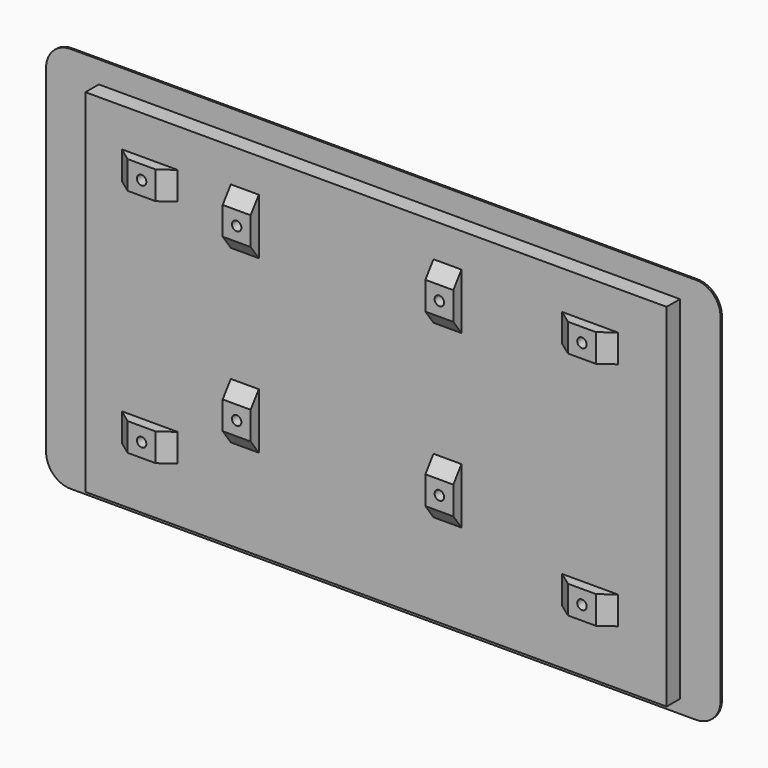
from build123d import *

# Parameters (mm, degrees)
F0_W     = 166.3
F0_H     = 100.7
F0_W_2   = 154.8
F0_H_2   = 87.4
F0_W_3   = 8
F0_H_3   = 8
F0_R     = 1.35
F1_DEPTH = 0.5
F2_DEPTH = 4.8
F3_DEPTH = 7.7
F4_SIZE2 = 2.89999
F4_SIZE  = 3.99999
F5_DEPTH = 0.51


# Not quite as in the source:
# - a fillet or chamfer is up to 0.001 mm smaller than in the source, because OpenCascade refuses the exact size


with BuildPart() as f1:
    # F0 (on Front) → F1 (new body)
    with BuildSketch(Plane.XZ):
        with BuildLine():
            Line((67.3, 73), (-111.7, 73))
            ThreePointArc((-111.7, 73), (-116.6497474683, 70.9497474683), (-118.7, 66))
            Line((-118.7, 66), (-118.7, -30.8))
            ThreePointArc((-118.7, -30.8), (-116.6497474683, -35.7497474683), (-111.7, -37.8))
            Line((-111.7, -37.8), (67.3, -37.8))
            ThreePointArc((67.3, -37.8), (72.2497474683, -35.7497474683), (74.3, -30.8))
            Line((74.3, -30.8), (74.3, 66))
            ThreePointArc((74.3, 66), (72.2497474683, 70.9497474683), (67.3, 73))
        make_face()
        with Locations((-20.45, 16.35)):
            Rectangle(F0_W, F0_H, mode=Mode.SUBTRACT)
        with Locations((-20.45, 16.35)):
            Rectangle(F0_W, F0_H)
        with Locations((-22.2, 18.6)):
            Rectangle(F0_W_2, F0_H_2, mode=Mode.SUBTRACT)
        with Locations((-22.2, 18.6)):
            Rectangle(F0_W_2, F0_H_2)
        with Locations((-85.2, -14.3)):
            Rectangle(F0_W_3, F0_H_3, mode=Mode.SUBTRACT)
        with Locations((-58, 0)):
            Rectangle(F0_W_3, F0_H_3, mode=Mode.SUBTRACT)
        with Locations((40.8, -14.3)):
            Rectangle(F0_W_3, F0_H_3, mode=Mode.SUBTRACT)
        Rectangle(F0_W_3, F0_H_3, mode=Mode.SUBTRACT)
        with Locations((-85.2, 51.7)):
            Rectangle(F0_W_3, F0_H_3, mode=Mode.SUBTRACT)
        with Locations((-58, 49)):
            Rectangle(F0_W_3, F0_H_3, mode=Mode.SUBTRACT)
        with Locations((0, 49)):
            Rectangle(F0_W_3, F0_H_3, mode=Mode.SUBTRACT)
        with Locations((40.8, 51.7)):
            Rectangle(F0_W_3, F0_H_3, mode=Mode.SUBTRACT)
        with Locations((-58, 49)):
            Rectangle(F0_W_3, F0_H_3)
        with Locations((-58, 49)):
            Circle(F0_R, mode=Mode.SUBTRACT)
        with Locations((-85.2, 51.7)):
            Rectangle(F0_W_3, F0_H_3)
        with Locations((-85.2, 51.7)):
            Circle(F0_R, mode=Mode.SUBTRACT)
        with Locations((40.8, 51.7)):
            Rectangle(F0_W_3, F0_H_3)
        with Locations((40.8, 51.7)):
            Circle(F0_R, mode=Mode.SUBTRACT)
        Rectangle(F0_W_3, F0_H_3)
        Circle(F0_R, mode=Mode.SUBTRACT)
        with Locations((40.8, -14.3)):
            Rectangle(F0_W_3, F0_H_3)
        with Locations((40.8, -14.3)):
            Circle(F0_R, mode=Mode.SUBTRACT)
        with Locations((0, 49)):
            Rectangle(F0_W_3, F0_H_3)
        with Locations((0, 49)):
            Circle(F0_R, mode=Mode.SUBTRACT)
        with Locations((-58, 0)):
            Rectangle(F0_W_3, F0_H_3)
        with Locations((-58, 0)):
            Circle(F0_R, mode=Mode.SUBTRACT)
        with Locations((-85.2, -14.3)):
            Rectangle(F0_W_3, F0_H_3)
        with Locations((-85.2, -14.3)):
            Circle(F0_R, mode=Mode.SUBTRACT)
        with Locations((0, 49)):
            Circle(F0_R)
        with Locations((40.8, 51.7)):
            Circle(F0_R)
        with Locations((40.8, -14.3)):
            Circle(F0_R)
        Circle(F0_R)
        with Locations((-58, 49)):
            Circle(F0_R)
        with Locations((-58, 0)):
            Circle(F0_R)
        with Locations((-85.2, 51.7)):
            Circle(F0_R)
        with Locations((-85.2, -14.3)):
            Circle(F0_R)
    extrude(amount=-F1_DEPTH)


with BuildPart() as f2:
    # F0 (on Front) → F2 (new body)
    with BuildSketch(Plane.XZ):
        with Locations((-20.45, 16.35)):
            Rectangle(F0_W, F0_H)
        with Locations((-22.2, 18.6)):
            Rectangle(F0_W_2, F0_H_2, mode=Mode.SUBTRACT)
        with Locations((-22.2, 18.6)):
            Rectangle(F0_W_2, F0_H_2)
        with Locations((-85.2, -14.3)):
            Rectangle(F0_W_3, F0_H_3, mode=Mode.SUBTRACT)
        with Locations((-58, 0)):
            Rectangle(F0_W_3, F0_H_3, mode=Mode.SUBTRACT)
        with Locations((40.8, -14.3)):
            Rectangle(F0_W_3, F0_H_3, mode=Mode.SUBTRACT)
        Rectangle(F0_W_3, F0_H_3, mode=Mode.SUBTRACT)
        with Locations((-85.2, 51.7)):
            Rectangle(F0_W_3, F0_H_3, mode=Mode.SUBTRACT)
        with Locations((-58, 49)):
            Rectangle(F0_W_3, F0_H_3, mode=Mode.SUBTRACT)
        with Locations((0, 49)):
            Rectangle(F0_W_3, F0_H_3, mode=Mode.SUBTRACT)
        with Locations((40.8, 51.7)):
            Rectangle(F0_W_3, F0_H_3, mode=Mode.SUBTRACT)
        with Locations((40.8, 51.7)):
            Rectangle(F0_W_3, F0_H_3)
        with Locations((40.8, 51.7)):
            Circle(F0_R, mode=Mode.SUBTRACT)
        with Locations((0, 49)):
            Rectangle(F0_W_3, F0_H_3)
        with Locations((0, 49)):
            Circle(F0_R, mode=Mode.SUBTRACT)
        with Locations((-58, 49)):
            Rectangle(F0_W_3, F0_H_3)
        with Locations((-58, 49)):
            Circle(F0_R, mode=Mode.SUBTRACT)
        with Locations((-85.2, 51.7)):
            Rectangle(F0_W_3, F0_H_3)
        with Locations((-85.2, 51.7)):
            Circle(F0_R, mode=Mode.SUBTRACT)
        with Locations((-58, 0)):
            Rectangle(F0_W_3, F0_H_3)
        with Locations((-58, 0)):
            Circle(F0_R, mode=Mode.SUBTRACT)
        with Locations((-85.2, -14.3)):
            Rectangle(F0_W_3, F0_H_3)
        with Locations((-85.2, -14.3)):
            Circle(F0_R, mode=Mode.SUBTRACT)
        Rectangle(F0_W_3, F0_H_3)
        Circle(F0_R, mode=Mode.SUBTRACT)
        with Locations((40.8, -14.3)):
            Rectangle(F0_W_3, F0_H_3)
        with Locations((40.8, -14.3)):
            Circle(F0_R, mode=Mode.SUBTRACT)
        with Locations((40.8, 51.7)):
            Circle(F0_R)
        with Locations((0, 49)):
            Circle(F0_R)
        with Locations((-58, 49)):
            Circle(F0_R)
        with Locations((-85.2, 51.7)):
            Circle(F0_R)
        with Locations((-58, 0)):
            Circle(F0_R)
        with Locations((-85.2, -14.3)):
            Circle(F0_R)
        Circle(F0_R)
        with Locations((40.8, -14.3)):
            Circle(F0_R)
    extrude(amount=F2_DEPTH)

    # F0 (on Front) → F3 (join)
    with BuildSketch(Plane.XZ):
        with Locations((-58, 49)):
            Rectangle(F0_W_3, F0_H_3)
        with Locations((-58, 49)):
            Circle(F0_R, mode=Mode.SUBTRACT)
        with Locations((0, 49)):
            Rectangle(F0_W_3, F0_H_3)
        with Locations((0, 49)):
            Circle(F0_R, mode=Mode.SUBTRACT)
        with Locations((40.8, 51.7)):
            Rectangle(F0_W_3, F0_H_3)
        with Locations((40.8, 51.7)):
            Circle(F0_R, mode=Mode.SUBTRACT)
        with Locations((40.8, -14.3)):
            Rectangle(F0_W_3, F0_H_3)
        with Locations((40.8, -14.3)):
            Circle(F0_R, mode=Mode.SUBTRACT)
        Rectangle(F0_W_3, F0_H_3)
        Circle(F0_R, mode=Mode.SUBTRACT)
        with Locations((-58, 0)):
            Rectangle(F0_W_3, F0_H_3)
        with Locations((-58, 0)):
            Circle(F0_R, mode=Mode.SUBTRACT)
        with Locations((-85.2, -14.3)):
            Rectangle(F0_W_3, F0_H_3)
        with Locations((-85.2, -14.3)):
            Circle(F0_R, mode=Mode.SUBTRACT)
        with Locations((-85.2, 51.7)):
            Rectangle(F0_W_3, F0_H_3)
        with Locations((-85.2, 51.7)):
            Circle(F0_R, mode=Mode.SUBTRACT)
    extrude(amount=F3_DEPTH)

    # F4 (size 4 and 2.9 in the source; OpenCascade refuses exactly that, so slightly less here)
    f4_edges = [f2.edges().sort_by_distance(p)[0] for p in [
        (-58, -4.8, 53),
        (-58, -4.8, 45),
        (-89.2, -4.8, 51.7),
        (-81.2, -4.8, 51.7),
        (0, -4.8, 45),
        (0, -4.8, -4),
        (44.8, -4.8, -14.3),
        (44.8, -4.8, 51.7),
        (-58, -4.8, -4),
        (-81.2, -4.8, -14.3),
        (-89.2, -4.8, -14.3),
        (36.8, -4.8, 51.7),
        (36.8, -4.8, -14.3),
        (0, -4.8, 53),
        (0, -4.8, 4),
        (-58, -4.8, 4),
    ]]
    chamfer(f4_edges, length=F4_SIZE, length2=F4_SIZE2)


with BuildPart() as f5:
    # F0 (on Front) → F5 (new body)
    with BuildSketch(Plane.XZ):
        with Locations((-22.2, 18.6)):
            Rectangle(F0_W_2, F0_H_2)
        with Locations((-85.2, -14.3)):
            Rectangle(F0_W_3, F0_H_3, mode=Mode.SUBTRACT)
        with Locations((-58, 0)):
            Rectangle(F0_W_3, F0_H_3, mode=Mode.SUBTRACT)
        with Locations((40.8, -14.3)):
            Rectangle(F0_W_3, F0_H_3, mode=Mode.SUBTRACT)
        Rectangle(F0_W_3, F0_H_3, mode=Mode.SUBTRACT)
        with Locations((-85.2, 51.7)):
            Rectangle(F0_W_3, F0_H_3, mode=Mode.SUBTRACT)
        with Locations((-58, 49)):
            Rectangle(F0_W_3, F0_H_3, mode=Mode.SUBTRACT)
        with Locations((0, 49)):
            Rectangle(F0_W_3, F0_H_3, mode=Mode.SUBTRACT)
        with Locations((40.8, 51.7)):
            Rectangle(F0_W_3, F0_H_3, mode=Mode.SUBTRACT)
        with Locations((40.8, 51.7)):
            Rectangle(F0_W_3, F0_H_3)
        with Locations((40.8, 51.7)):
            Circle(F0_R, mode=Mode.SUBTRACT)
        with Locations((40.8, -14.3)):
            Rectangle(F0_W_3, F0_H_3)
        with Locations((40.8, -14.3)):
            Circle(F0_R, mode=Mode.SUBTRACT)
        with Locations((0, 49)):
            Rectangle(F0_W_3, F0_H_3)
        with Locations((0, 49)):
            Circle(F0_R, mode=Mode.SUBTRACT)
        with Locations((-58, 49)):
            Rectangle(F0_W_3, F0_H_3)
        with Locations((-58, 49)):
            Circle(F0_R, mode=Mode.SUBTRACT)
        with Locations((-85.2, 51.7)):
            Rectangle(F0_W_3, F0_H_3)
        with Locations((-85.2, 51.7)):
            Circle(F0_R, mode=Mode.SUBTRACT)
        with Locations((-58, 0)):
            Rectangle(F0_W_3, F0_H_3)
        with Locations((-58, 0)):
            Circle(F0_R, mode=Mode.SUBTRACT)
        with Locations((-85.2, -14.3)):
            Rectangle(F0_W_3, F0_H_3)
        with Locations((-85.2, -14.3)):
            Circle(F0_R, mode=Mode.SUBTRACT)
        Rectangle(F0_W_3, F0_H_3)
        Circle(F0_R, mode=Mode.SUBTRACT)
        with Locations((40.8, 51.7)):
            Circle(F0_R)
        with Locations((40.8, -14.3)):
            Circle(F0_R)
        Circle(F0_R)
        with Locations((0, 49)):
            Circle(F0_R)
        with Locations((-58, 49)):
            Circle(F0_R)
        with Locations((-58, 0)):
            Circle(F0_R)
        with Locations((-85.2, 51.7)):
            Circle(F0_R)
        with Locations((-85.2, -14.3)):
            Circle(F0_R)
    extrude(amount=-F5_DEPTH)


solid = Compound([f1.part, f2.part, f5.part])
